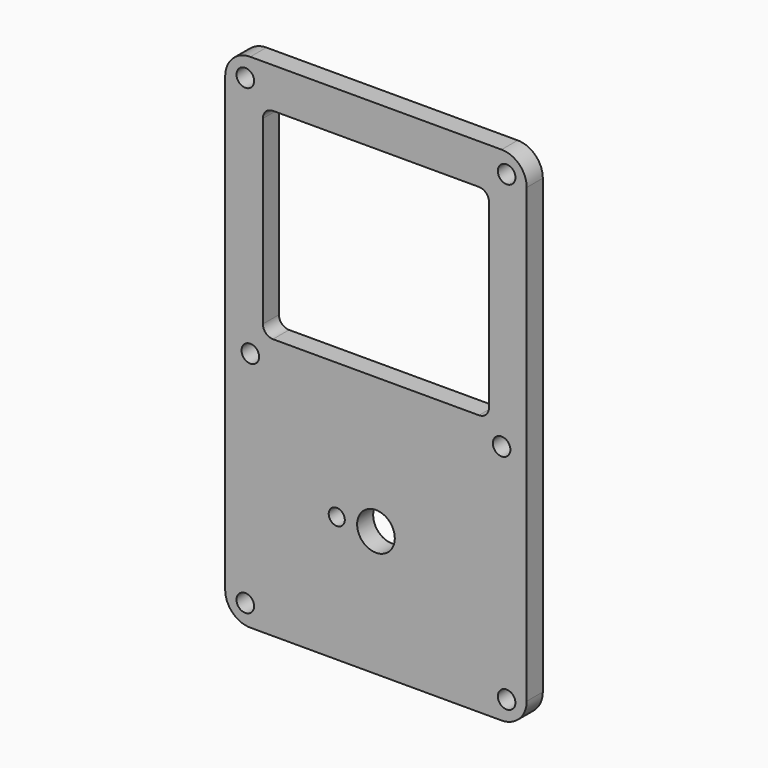
from build123d import *

# Parameters (mm, degrees)
F0_W      = 60
F0_H      = 100
F0_W_2    = 45
F0_H_2    = 40
F1_DEPTH  = 4
F3_D      = 3.5
F3_DEPTH  = 25
F3_TIP    = 1.0515060833
F5_R      = 5
F6_R      = 2
F8_D      = 3.5
F8_DEPTH  = 25
F8_TIP    = 1.0515060833
F4_R      = 3.75
F4_R_2    = 1.6
F9_DEPTH  = 25
F10_DEPTH = 25


# Not quite as in the source:
# - a feature names something its author has since deleted; it is built from what else it names


with BuildPart() as f1:
    # F0 (on Front) → F1 (new body)
    with BuildSketch(Plane.XZ):
        Rectangle(F0_W, F0_H)
        with Locations((0, 22)):
            Rectangle(F0_W_2, F0_H_2, mode=Mode.SUBTRACT)
    extrude(amount=F1_DEPTH)

    # F3
    with Locations(Plane.XZ.offset(4)):
        with Locations((-26, 46), (26, 46), (26, -46), (-26, -46)):
            Hole(F3_D / 2, depth=F3_DEPTH)
            with Locations((0, 0, -(F3_DEPTH + F3_TIP / 2))):  # 118° drill point
                Cone(0, F3_D / 2, F3_TIP, mode=Mode.SUBTRACT)

    # F5
    f5_edges = [f1.edges().sort_by_distance(p)[0] for p in [
        (-30, -2, 50),
        (-30, -2, -50),
        (30, -2, -50),
        (30, -2, 50),
    ]]
    fillet(f5_edges, radius=F5_R)

    # F6
    f6_edges = [f1.edges().sort_by_distance(p)[0] for p in [
        (-22.5, -2, 2),
        (-22.5, -2, 42),
        (22.5, -2, 42),
        (22.5, -2, 2),
    ]]
    fillet(f6_edges, radius=F6_R)

    # F8
    with Locations(Plane.XZ.offset(4)):
        with Locations((-25, -2), (25, -2)):
            Hole(F8_D / 2, depth=F8_DEPTH)
            with Locations((0, 0, -(F8_DEPTH + F8_TIP / 2))):  # 118° drill point
                Cone(0, F8_D / 2, F8_TIP, mode=Mode.SUBTRACT)

    # F4 (on face) → F9 (cut)
    with BuildSketch(Plane.XZ.offset(4)):
        with Locations((0, -25)):
            Circle(F4_R)
        with Locations((-7.8, -25)):
            Circle(F4_R_2)
    extrude(amount=-F9_DEPTH, mode=Mode.SUBTRACT)

    # F4 (on face) → F10 (cut)
    with BuildSketch(Plane.XZ.offset(4)):
        with Locations((0, -25)):
            Circle(F4_R)
        with Locations((-7.8, -25)):
            Circle(F4_R_2)
    extrude(amount=-F10_DEPTH, mode=Mode.SUBTRACT)


solid = f1.part
